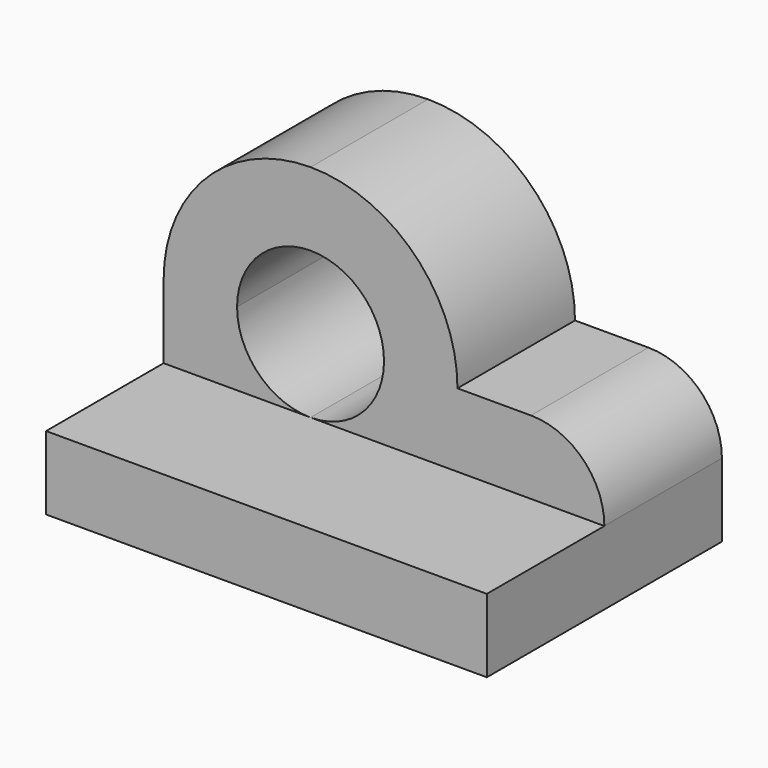
from build123d import *

# Parameters (mm, degrees)
F0_W     = 60
F0_H     = 40
F1_DEPTH = 40
F2_W     = 60
F2_H     = 20
F3_DEPTH = 30
F4_R     = 10
F5_DEPTH = 20
F7_DEPTH = 20
F9_DEPTH = 20


with BuildPart() as f1:
    # F0 (on Top) → F1 (new body)
    with BuildSketch(Plane.XY):
        with Locations((30, 20)):
            Rectangle(F0_W, F0_H)
    extrude(amount=F1_DEPTH)

    # F2 (on face) → F3 (cut)
    with BuildSketch(Plane.XY.offset(40)):
        with Locations((30, 10)):
            Rectangle(F2_W, F2_H)
    extrude(amount=-F3_DEPTH, mode=Mode.SUBTRACT)

    # F4 (on face) → F5 (join)
    with BuildSketch(Plane.XZ.offset(-20)):
        with Locations((17.3286311328, 20.5947589129)):
            Circle(F4_R)
    extrude(amount=-F5_DEPTH)

    # F6 (on face) → F7 (cut)
    with BuildSketch(Plane.XZ.offset(-20)):
        with BuildLine():
            ThreePointArc((30, 20), (20, 30), (10, 20))
            Line((10, 20), (20, 20))
            Line((20, 20), (30, 20))
        make_face()
        with BuildLine():
            ThreePointArc((10, 20), (12.9289321881, 12.9289321881), (20, 10))
            ThreePointArc((20, 10), (27.0710678119, 12.9289321881), (30, 20))
            Line((30, 20), (20, 20))
            Line((20, 20), (10, 20))
        make_face()
        with BuildLine():
            Line((0, 40), (0, 20))
            ThreePointArc((0, 20), (5.8578643763, 34.1421356237), (20, 40))
            Line((20, 40), (0, 40))
        make_face()
        with BuildLine():
            Line((60, 40), (20, 40))
            ThreePointArc((20, 40), (34.1421356237, 34.1421356237), (40, 20))
            Line((40, 20), (50, 20))
            Line((50, 20), (60, 20))
            Line((60, 20), (60, 40))
        make_face()
    extrude(amount=-F7_DEPTH, mode=Mode.SUBTRACT)

    # F8 (on face) → F9 (cut)
    with BuildSketch(Plane.XZ.offset(-20)):
        with BuildLine():
            ThreePointArc((50, 20), (57.0710678119, 17.0710678119), (60, 10))
            Line((60, 10), (60, 20))
            Line((60, 20), (50, 20))
        make_face()
    extrude(amount=-F9_DEPTH, mode=Mode.SUBTRACT)


solid = f1.part
